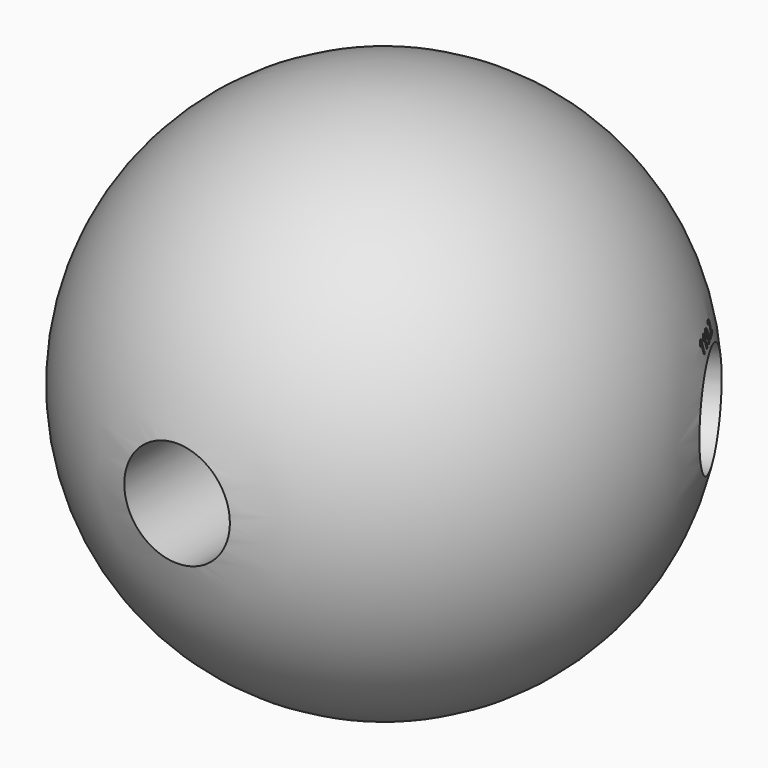
from build123d import *

# Parameters (mm, degrees)
F4_R          = 3.175
F5_DEPTH      = 25.4
F7_ANGLE      = 119.2
F8_ANGLE      = -119.2
F10_TEXT_SIZE = 1.1681194236
F11_DEPTH     = 2.413
F13_TEXT_SIZE = 1.0501690364
F14_DEPTH     = 2.1082


# Not quite as in the source:
# - Text() gives the source's letters only with a copy of the font that has no kerning and outlines rounded to 1/6400 em; it was checked with that copy


with BuildPart() as f2:
    # F0 (on Front) → F2 (revolve)
    with BuildSketch(Plane.XZ):
        with BuildLine():
            Line((0, -15.875), (0, 15.875))
            ThreePointArc((0, 15.875), (-15.875, 0), (0, -15.875))
        make_face()
    revolve(axis=Axis((0, 0, 0), (0, 0, 1)))

    # F10 (on offset) → F11 (cut)
    with BuildSketch(Plane(origin=(-14.4341157165, 8.0669546077, 0), x_dir=(-0.4878596591, -0.8729220773, 0), z_dir=(-0.8729220773, 0.4878596591, 0))):
        with Locations((-1.6862096963, 3.6194035783)):
            Text('119.2', F10_TEXT_SIZE, font='Open Sans', font_style=FontStyle.BOLD, text_align=(TextAlign.LEFT, TextAlign.BOTTOM))
    extrude(amount=-F11_DEPTH, mode=Mode.SUBTRACT)

    # F13 (on offset) → F14 (cut)
    with BuildSketch(Plane(origin=(14.5006323788, 8.1041295137, 0), x_dir=(-0.4878596591, 0.8729220773, 0), z_dir=(0.8729220773, 0.4878596591, 0))):
        with Locations((-1.4730878174, 3.4820353612)):
            Text('119.2', F13_TEXT_SIZE, font='Open Sans', font_style=FontStyle.BOLD, text_align=(TextAlign.LEFT, TextAlign.BOTTOM))
    extrude(amount=-F14_DEPTH, mode=Mode.SUBTRACT)


with BuildPart() as f5:
    # F4 (on offset) → F5 (new body)
    with BuildSketch(Plane.XZ.offset(6.35)):
        Circle(F4_R)
    extrude(amount=F5_DEPTH)


with BuildPart() as f7_1:
    # F7: copy of F5
    add(f5.part.rotate(Axis((0, 0, 6.8211313337), (0, 0, -1)), F7_ANGLE))


with BuildPart() as f8_1:
    # F8: copy of F5
    add(f5.part.rotate(Axis((0, 0, 6.8211313337), (0, 0, -1)), F8_ANGLE))


with BuildPart() as f2_1:
    add(f2.part)

    # F15: cut F7_1
    add(f7_1.part, mode=Mode.SUBTRACT)

    # F16: cut F8_1
    add(f8_1.part, mode=Mode.SUBTRACT)

    # F17: cut F5
    add(f5.part, mode=Mode.SUBTRACT)


solid = f2_1.part
